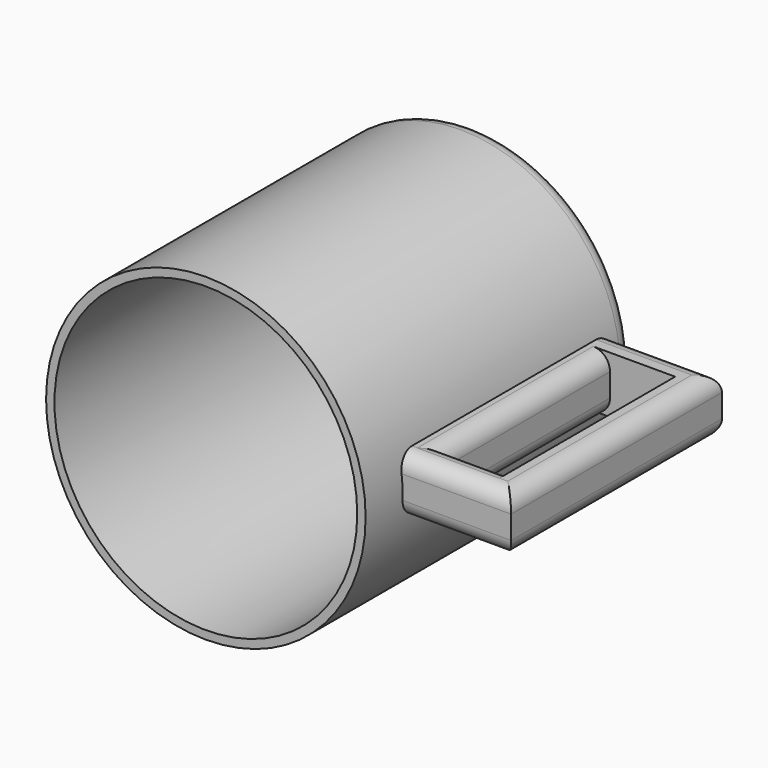
from build123d import *

# Parameters (mm, degrees)
F0_R         = 47.6611087375
F1_DEPTH     = 100
F2_T         = -2.5
F4_W         = 78.6115438677
F4_H         = 16.9129944406
F6_W         = 19.4371528924
F6_H         = 60.759909451
F7_DEPTH     = 25
F8_T1_DEPTH  = 57.743928854
F8_T3_DEPTH  = 58.5584052808
F8_T5_DEPTH  = 103.6115438677
F8_T7_DEPTH  = 60.759909451
F8_T9_DEPTH  = 19.4371528924
F8_T15_DEPTH = 73.259909451
F8_T20_DEPTH = 31.9371528924
F8_S22_R     = 47.6611087375
F8_T23_DEPTH = 18
F9_R         = 5


# Not quite as in the source:
# - a fillet or chamfer that OpenCascade refuses, or shapes differently, is made with other operations: its cross-section is extruded or revolved along the edge and cut away or added


with BuildPart() as f1:
    # F0 (on Front) → F1 (new body)
    with BuildSketch(Plane.XZ):
        Circle(F0_R)
    extrude(amount=F1_DEPTH)

    # F2
    f2_openings = [f1.faces().sort_by_distance(p)[0] for p in [
        (0, -100, 0),
    ]]
    offset(amount=F2_T, openings=f2_openings)


with BuildPart() as f5:
    # F4 (on offset) → F5 (new body, up to the next surface of F1)
    with BuildSketch(Plane.YZ.offset(80)):
        with Locations((-46.8722551595, 2.2560919169)):
            Rectangle(F4_W, F4_H)
    extrude(until=Until.NEXT, target=f1.part, dir=(-1, 0, 0))

    # F6 (on face) → F7 (cut)
    with BuildSketch(Plane.XY.offset(10.7125891373)):
        with Locations((62.8032963723, -46.0315085948)):
            Rectangle(F6_W, F6_H)
    extrude(amount=-F7_DEPTH, mode=Mode.SUBTRACT)

    # F8: fillet of radius 5 on 9 edges, made by hand

    # F8_s2 → F8_t1 (cut)
    with BuildSketch(Plane.YZ.offset(34.756071146)):
        with BuildLine():
            ThreePointArc((-86.1780270934, -1.2004053034), (-84.7135609993, -4.7359392093), (-81.1780270934, -6.2004053034))
            Line((-81.1780270934, -6.2004053034), (-86.1780270934, -6.2004053034))
            Line((-86.1780270934, -6.2004053034), (-86.1780270934, -1.2004053034))
        make_face()
        with BuildLine():
            ThreePointArc((-12.5664832257, -6.2004053034), (-9.0309493197, -4.7359392093), (-7.5664832257, -1.2004053034))
            Line((-7.5664832257, -1.2004053034), (-7.5664832257, -6.2004053034))
            Line((-7.5664832257, -6.2004053034), (-12.5664832257, -6.2004053034))
        make_face()
    extrude(amount=F8_T1_DEPTH, mode=Mode.SUBTRACT)

    # F8_s4 → F8_t3 (cut)
    with BuildSketch(Plane.YZ.offset(33.9415947192)):
        with BuildLine():
            ThreePointArc((-86.1780270934, 5.7125891373), (-84.7135609993, 9.2481230432), (-81.1780270934, 10.7125891373))
            Line((-81.1780270934, 10.7125891373), (-86.1780270934, 10.7125891373))
            Line((-86.1780270934, 10.7125891373), (-86.1780270934, 5.7125891373))
        make_face()
        with BuildLine():
            ThreePointArc((-7.5664832257, 5.7125891373), (-9.0309493197, 9.2481230432), (-12.5664832257, 10.7125891373))
            Line((-12.5664832257, 10.7125891373), (-7.5664832257, 10.7125891373))
            Line((-7.5664832257, 10.7125891373), (-7.5664832257, 5.7125891373))
        make_face()
    extrude(amount=F8_T3_DEPTH, mode=Mode.SUBTRACT)

    # F8_s6 → F8_t5 (cut)
    with BuildSketch(Plane.XZ.offset(-4.9335167743)):
        with BuildLine():
            ThreePointArc((75, 10.7125891373), (78.5355339059, 9.2481230432), (80, 5.7125891373))
            Line((80, 5.7125891373), (80, 10.7125891373))
            Line((80, 10.7125891373), (75, 10.7125891373))
        make_face()
        with BuildLine():
            ThreePointArc((75, -6.2004053034), (78.5355339059, -4.7359392093), (80, -1.2004053034))
            Line((80, -1.2004053034), (80, -6.2004053034))
            Line((80, -6.2004053034), (75, -6.2004053034))
        make_face()
    extrude(amount=F8_T5_DEPTH, mode=Mode.SUBTRACT)

    # F8_s8 → F8_t7 (cut)
    with BuildSketch(Plane.XZ.offset(15.6515538692)):
        with BuildLine():
            ThreePointArc((53.0847199261, 5.7125891373), (51.6202538321, 9.2481230432), (48.0847199261, 10.7125891373))
            Line((48.0847199261, 10.7125891373), (53.0847199261, 10.7125891373))
            Line((53.0847199261, 10.7125891373), (53.0847199261, 5.7125891373))
        make_face()
        with BuildLine():
            ThreePointArc((48.0847199261, -6.2004053034), (51.6202538321, -4.7359392093), (53.0847199261, -1.2004053034))
            Line((53.0847199261, -1.2004053034), (53.0847199261, -6.2004053034))
            Line((53.0847199261, -6.2004053034), (48.0847199261, -6.2004053034))
        make_face()
    extrude(amount=F8_T7_DEPTH, mode=Mode.SUBTRACT)

    # F8_s10 → F8_t9 (cut)
    with BuildSketch(Plane.YZ.offset(53.0847199261)):
        with BuildLine():
            ThreePointArc((-76.4114633203, 5.7125891373), (-77.8759294143, 9.2481230432), (-81.4114633203, 10.7125891373))
            Line((-81.4114633203, 10.7125891373), (-76.4114633203, 10.7125891373))
            Line((-76.4114633203, 10.7125891373), (-76.4114633203, 5.7125891373))
        make_face()
    extrude(amount=F8_T9_DEPTH, mode=Mode.SUBTRACT)


with BuildPart() as f8_tool13:
    # F8_s14 → F8_t15 (new body)
    with BuildSketch(Plane.XZ.offset(15.6515538692)):
        with BuildLine():
            ThreePointArc((53.0847199261, 5.7125891373), (51.6202538321, 9.2481230432), (48.0847199261, 10.7125891373))
            Line((48.0847199261, 10.7125891373), (53.0847199261, 10.7125891373))
            Line((53.0847199261, 10.7125891373), (53.0847199261, 5.7125891373))
        make_face()
    extrude(amount=F8_T15_DEPTH)

    split(bisect_by=Plane.XZ.offset(86.1780270934), keep=Keep.BOTTOM)

    split(bisect_by=Plane.XZ.offset(76.4114633203), keep=Keep.TOP)


with BuildPart() as f8_tool18:
    # F8_s19 → F8_t20 (new body)
    with BuildSketch(Plane.YZ.offset(40.5847199261)):
        with BuildLine():
            ThreePointArc((-76.4114633203, 5.7125891373), (-77.8759294143, 9.2481230432), (-81.4114633203, 10.7125891373))
            Line((-81.4114633203, 10.7125891373), (-76.4114633203, 10.7125891373))
            Line((-76.4114633203, 10.7125891373), (-76.4114633203, 5.7125891373))
        make_face()
    extrude(amount=F8_T20_DEPTH)

    split(bisect_by=Plane.YZ.offset(53.0847199261), keep=Keep.BOTTOM)

    # F8_s22 → F8_t23 (cut, symmetric)
    with BuildSketch(Plane.XZ.offset(78.9)):
        Circle(F8_S22_R)
    extrude(amount=F8_T23_DEPTH, both=True, mode=Mode.SUBTRACT)


with BuildPart() as f8_tool13_1:
    add(f8_tool13.part)

    # F8_t24: intersect F8_tool18
    add(f8_tool18.part, mode=Mode.INTERSECT)


with BuildPart() as f5_1:
    add(f5.part)

    # F8_t11: cut F8_tool13
    add(f8_tool13_1.part, mode=Mode.SUBTRACT)


with BuildPart() as f1_1:
    add(f1.part)

    # F9
    f9_edges = [f1_1.edges().sort_by_distance(p)[0] for p in [
        (-47.661109, 0, 0),
    ]]
    fillet(f9_edges, radius=F9_R)


solid = Compound([f5_1.part, f1_1.part])
